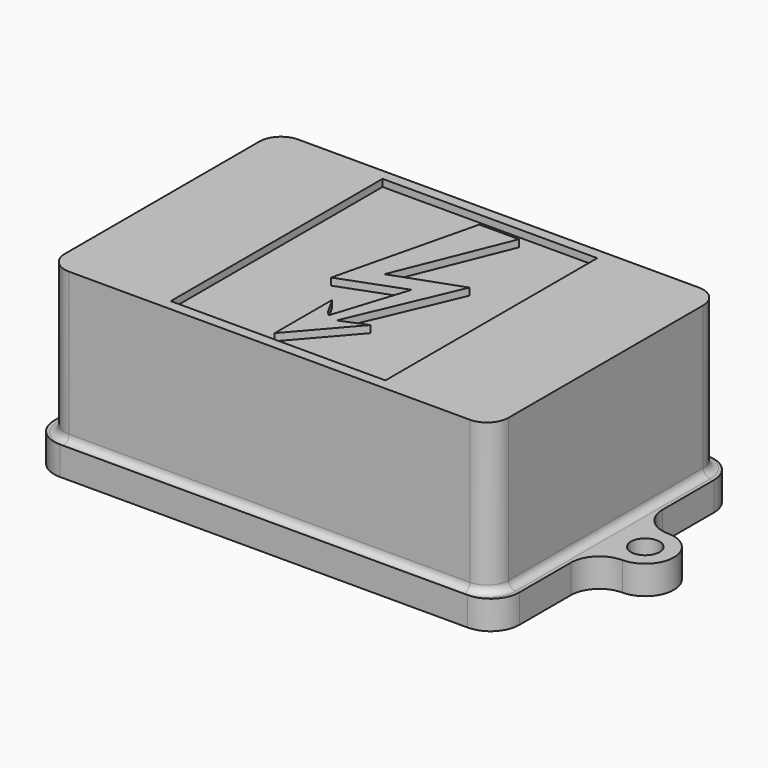
from build123d import *

# Parameters (mm, degrees)
F0_R     = 2
F1_DEPTH = 4
F3_DEPTH = 25
F4_R     = 0.99999
F5_DEPTH = 23
F7_START = 24
F6_W     = 30
F6_H     = 37
F7_DEPTH = 6
F9_DEPTH = 25


# Not quite as in the source:
# - a fillet or chamfer is up to 0.001 mm smaller than in the source, because OpenCascade refuses the exact size


with BuildPart() as f1:
    # F0 (on Top) → F1 (new body)
    with BuildSketch(Plane.XY):
        with BuildLine():
            Line((28.5, 21), (-28.5, 21))
            ThreePointArc((-28.5, 21), (-31.3284271247, 19.8284271247), (-32.5, 17))
            Line((-32.5, 17), (-32.5, 8))
            ThreePointArc((-32.5, 8), (-33.6715728753, 5.1715728753), (-36.5, 4))
            ThreePointArc((-36.5, 4), (-40.5, 0), (-36.5, -4))
            ThreePointArc((-36.5, -4), (-33.6715728753, -5.1715728753), (-32.5, -8))
            Line((-32.5, -8), (-32.5, -17))
            ThreePointArc((-32.5, -17), (-31.3284271247, -19.8284271247), (-28.5, -21))
            Line((-28.5, -21), (28.5, -21))
            ThreePointArc((28.5, -21), (31.3284271247, -19.8284271247), (32.5, -17))
            Line((32.5, -17), (32.5, -8))
            ThreePointArc((32.5, -8), (33.6715728753, -5.1715728753), (36.5, -4))
            ThreePointArc((36.5, -4), (40.5, 0), (36.5, 4))
            ThreePointArc((36.5, 4), (33.6715728753, 5.1715728753), (32.5, 8))
            Line((32.5, 8), (32.5, 17))
            ThreePointArc((32.5, 17), (31.3284271247, 19.8284271247), (28.5, 21))
        make_face()
        with Locations((-36.5, 0)):
            Circle(F0_R, mode=Mode.SUBTRACT)
        with BuildLine():
            ThreePointArc((29.5, -16), (28.9142135624, -17.4142135624), (27.5, -18))
            Line((27.5, -18), (-27.5, -18))
            ThreePointArc((-27.5, -18), (-28.9142135624, -17.4142135624), (-29.5, -16))
            Line((-29.5, -16), (-29.5, 16))
            ThreePointArc((-29.5, 16), (-28.9142135624, 17.4142135624), (-27.5, 18))
            Line((-27.5, 18), (27.5, 18))
            ThreePointArc((27.5, 18), (28.9142135624, 17.4142135624), (29.5, 16))
            Line((29.5, 16), (29.5, -16))
        make_face(mode=Mode.SUBTRACT)
        with Locations((36.5, 0)):
            Circle(F0_R, mode=Mode.SUBTRACT)
    extrude(amount=F1_DEPTH)

    # F2 (on Top) → F3 (join)
    with BuildSketch(Plane.XY):
        with BuildLine():
            Line((28, 20), (-28, 20))
            ThreePointArc((-28, 20), (-30.1213203436, 19.1213203436), (-31, 17))
            Line((-31, 17), (-31, -17))
            ThreePointArc((-31, -17), (-30.1213203436, -19.1213203436), (-28, -20))
            Line((-28, -20), (28, -20))
            ThreePointArc((28, -20), (30.1213203436, -19.1213203436), (31, -17))
            Line((31, -17), (31, 17))
            ThreePointArc((31, 17), (30.1213203436, 19.1213203436), (28, 20))
        make_face()
    extrude(amount=F3_DEPTH)

    # F4 (radius 1 in the source; OpenCascade refuses exactly that, so slightly less here)
    f4_edges = [f1.edges().sort_by_distance(p)[0] for p in [
        (0, -20, 4),
        (30.12132, -19.12132, 4),
    ]]
    fillet(f4_edges, radius=F4_R)

    # F0 (on Top) → F5 (cut)
    with BuildSketch(Plane.XY):
        with BuildLine():
            Line((-27.5, -18), (27.5, -18))
            ThreePointArc((27.5, -18), (28.9142135624, -17.4142135624), (29.5, -16))
            Line((29.5, -16), (29.5, 16))
            ThreePointArc((29.5, 16), (28.9142135624, 17.4142135624), (27.5, 18))
            Line((27.5, 18), (-27.5, 18))
            ThreePointArc((-27.5, 18), (-28.9142135624, 17.4142135624), (-29.5, 16))
            Line((-29.5, 16), (-29.5, -16))
            ThreePointArc((-29.5, -16), (-28.9142135624, -17.4142135624), (-27.5, -18))
        make_face()
    extrude(amount=F5_DEPTH, mode=Mode.SUBTRACT)

    # F6 (on Top) → F7 (cut)
    with BuildSketch(Plane.XY.offset(F7_START)):
        Rectangle(F6_W, F6_H)
        Polygon((-4.8068542965, -3.2168254256), (0, 16.6418794543), (5.5426517501, 16.6418794543), (-0.7649944164, 1.0344976326), (8.4538720548, 4.3500550091), (1.9844917115, -10.7721220702), (5.5426517501, -9.3165114522), (-1.4119322877, -17.3223689198), (-1.4119322877, -7.2948294692), (0, -9.8017146811), (0.5527317408, -10.3439353406), (3.8597108796, 0), align=None, mode=Mode.SUBTRACT)
    extrude(amount=F7_DEPTH, mode=Mode.SUBTRACT)

    # F8 (on Front) → F9 (cut)
    with BuildSketch(Plane.XZ):
        with BuildLine():
            Line((3.1964714846, -4.5143875896), (2.9989856559, 3.0780066406))
            ThreePointArc((2.9989856559, 3.0780066406), (-0.0784155915, 5.9989749907), (-2.9989642698, 2.921175459))
            Line((-2.9989642698, 2.921175459), (-2.8035285154, -4.5143875896))
            Line((-2.8035285154, -4.5143875896), (3.1964714846, -4.5143875896))
        make_face()
    extrude(amount=-F9_DEPTH, mode=Mode.SUBTRACT)


solid = f1.part
